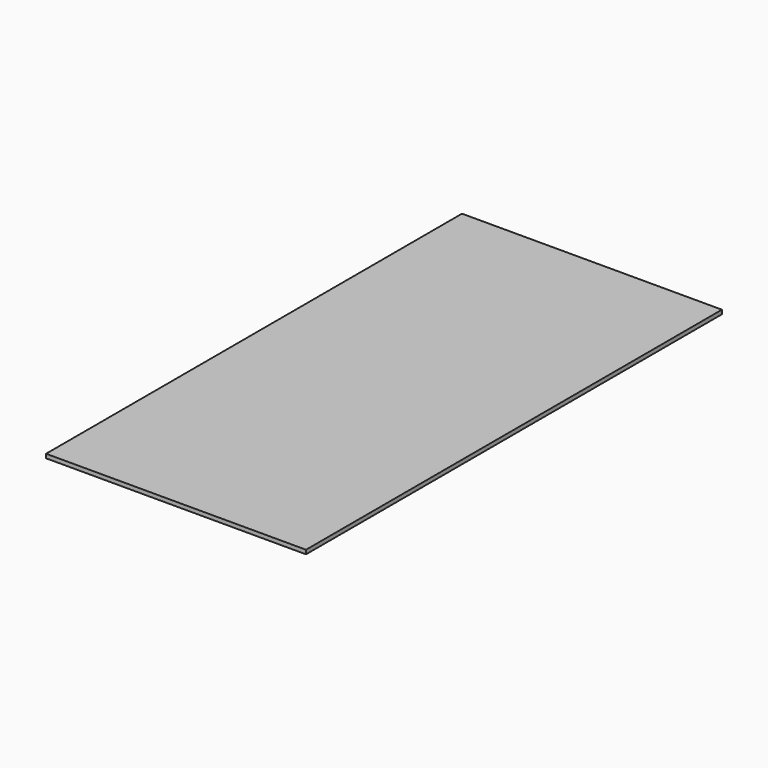
from build123d import *

# Parameters (mm, degrees)
F0_W     = 1219.2
F0_H     = 2438.4
F1_DEPTH = 19.05


# Not quite as in the source:
# - a length typed as a fraction of an inch, garbled in the dataset ("3 / 203.2 mm" for 3/8 in), is restored


with BuildPart() as f1:
    # F0 (on Top) → F1 (new body)
    with BuildSketch(Plane.XY):
        with Locations((1.5510842204, 362.1038203986)):
            Rectangle(F0_W, F0_H)
    extrude(amount=F1_DEPTH)


solid = f1.part
